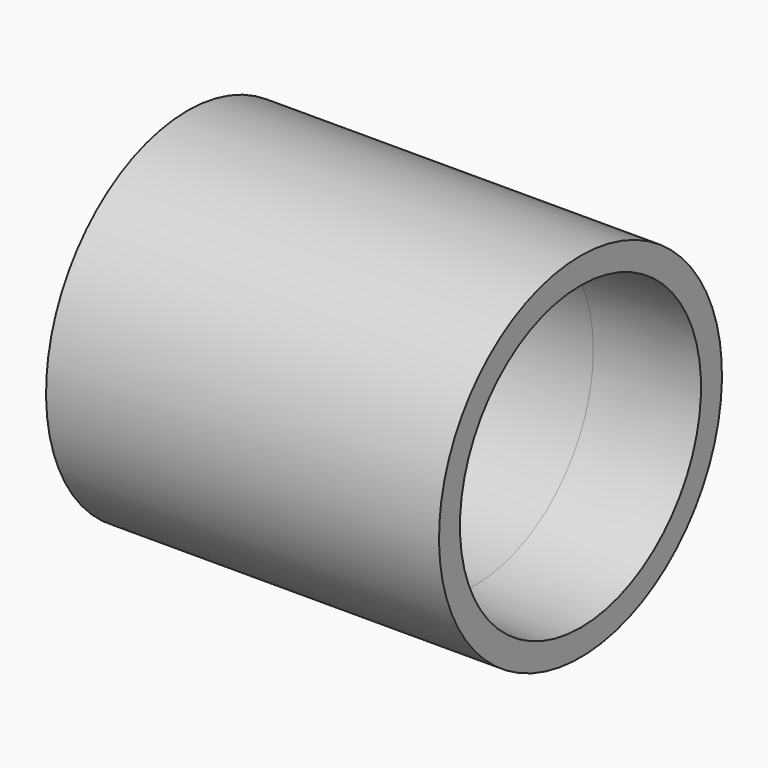
from build123d import *


# Not quite as in the source:
# - ends of sketch curves that miss each other by under 0.0002 mm in the source are joined


with BuildPart() as f1:
    # F0 (on Front) → F1 (revolve)
    with BuildSketch(Plane.XZ):
        Polygon((34.999999978, 67.5), (-75, 67.5), (-75, 56.125), (34.9996260565, 56.125), align=None)
        Polygon((75, 67.5), (34.999999978, 67.5), (34.9996260565, 56.125), (74.9996715909, 57.5095335858), align=None)
    revolve(axis=Axis((0, 0, 0), (1, 0, 0)))


solid = f1.part
